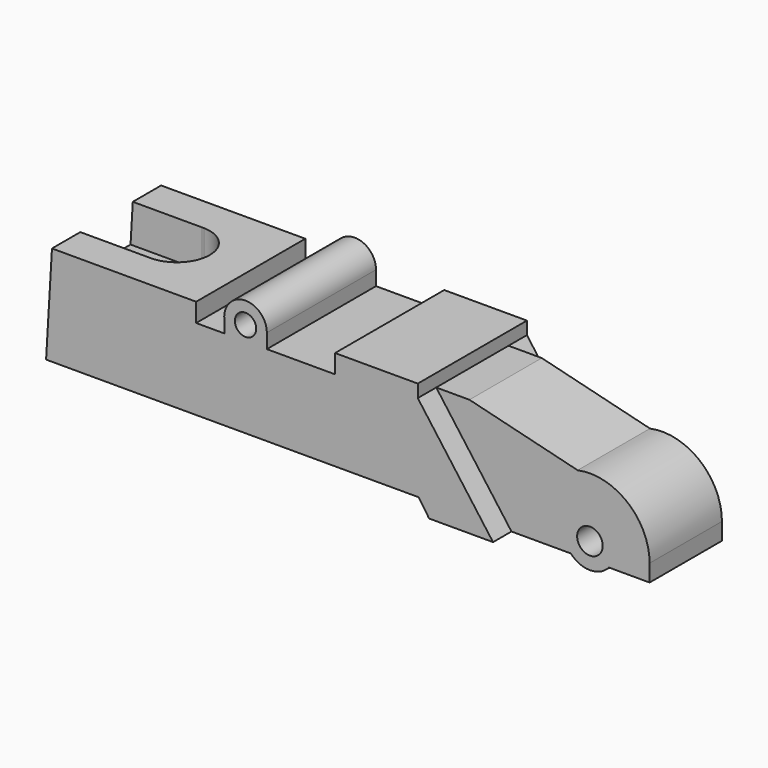
from build123d import *

# Parameters (mm, degrees)
F1_DEPTH  = 16
F2_R      = 1.5
F2_R_2    = 1.25
F3_DEPTH  = 16.001
F5_DEPTH  = 2.7
F8_DEPTH  = 14.501
F9_DEPTH  = 25
F11_DEPTH = 4.5


# Not quite as in the source:
# - a pattern or mirror of a feature is missing from the dataset's text; its kind, count and spacing are read off the source's solid


with BuildPart() as f1:
    # F0 (on Front) → F1 (new body)
    with BuildSketch(Plane.XZ):
        with BuildLine():
            Line((0.6909776407, 11.7), (0, 0))
            Line((0, 0), (43.7, 0))
            Line((43.7, 0), (44.92, -1.8))
            Line((44.92, -1.8), (59.3839320225, -1.8))
            ThreePointArc((59.3839320225, -1.8), (61.62, -2.8), (63.8560679775, -1.8))
            Line((63.8560679775, -1.8), (68.62, -1.8))
            Line((68.62, -1.8), (68.62, 0.2))
            ThreePointArc((68.62, 0.2), (66.0308120163, 5.6355070929), (60.1786464695, 7.05))
            Line((60.1786464695, 7.05), (47.4909776407, 10.2))
            Line((47.4909776407, 10.2), (43.5909776407, 10.2))
            Line((43.5909776407, 10.2), (43.5909776407, 11.7))
            Line((43.5909776407, 11.7), (33.8909776407, 11.7))
            Line((33.8909776407, 11.7), (33.8909776407, 9.5))
            Line((33.8909776407, 9.5), (25.8909776407, 9.5))
            Line((25.8909776407, 9.5), (25.8909776407, 11.2))
            ThreePointArc((25.8909776407, 11.2), (23.2847799515, 13.6977433917), (20.9, 10.9877963389))
            Line((20.9, 10.9877963389), (20.9, 9.5))
            Line((20.9, 9.5), (17.6, 9.5))
            Line((17.6, 9.5), (17.6, 11.7))
            Line((17.6, 11.7), (0.6909776407, 11.7))
        make_face()
    extrude(amount=F1_DEPTH)

    # F2 (on face) → F3 (cut, through all)
    with BuildSketch(Plane.XZ.offset(16)):
        with Locations((61.62, 0.2)):
            Circle(F2_R)
        with Locations((23.3909776407, 11.2)):
            Circle(F2_R_2)
    extrude(amount=-F3_DEPTH, mode=Mode.SUBTRACT)

    # F4 (on face) → F5 (cut)
    with BuildSketch(Plane.XZ.offset(16)):
        Polygon((69.0573006868, 10.2), (43.5909776407, 10.2), (52.42, -1.8), (58.7147176266, -4.3849991634), (70.332378149, -4.3849991634), align=None)
    f5 = extrude(amount=-F5_DEPTH, mode=Mode.SUBTRACT)

    # F5_copies: F5 across plane
    add(f5.mirror(Plane.ZX.offset(-8)), mode=Mode.SUBTRACT)

    # F7 (on face) → F8 (cut, through all)
    with BuildSketch(Plane.XY.offset(11.7)):
        with BuildLine():
            Line((8.9409776407, -5.75), (0.6909776407, -5.75))
            Line((0.6909776407, -5.75), (0.6909776407, -10.25))
            Line((0.6909776407, -10.25), (8.9409776407, -10.25))
            ThreePointArc((8.9409776407, -10.25), (11.1909776407, -8), (8.9409776407, -5.75))
        make_face()
    extrude(amount=-F8_DEPTH, mode=Mode.SUBTRACT)

    # F7 (on face) → F9 (cut)
    with BuildSketch(Plane.XY.offset(11.7)):
        with BuildLine():
            Line((8.9409776407, -5.75), (0.6909776407, -5.75))
            Line((0.6909776407, -5.75), (-0.8989692941, -5.75))
            Line((-0.8989692941, -5.75), (-0.8989692941, -10.25))
            Line((-0.8989692941, -10.25), (0.6909776407, -10.25))
            Line((0.6909776407, -10.25), (8.9409776407, -10.25))
            ThreePointArc((8.9409776407, -10.25), (11.1909776407, -8), (8.9409776407, -5.75))
        make_face()
    extrude(amount=-F9_DEPTH, mode=Mode.SUBTRACT)

    # F10 (on face) → F11 (cut)
    with BuildSketch(Plane.XY.offset(11.7)):
        with BuildLine():
            ThreePointArc((9.0590238842, -11.8481898452), (11.7047592925, -10.6803005393), (12.7909776407, -8))
            ThreePointArc((12.7909776407, -8), (11.7048621847, -5.3198055617), (9.0593193409, -4.1518192296))
            Line((9.0593193409, -4.1518192296), (8.8226359404, -4.1518192296))
            ThreePointArc((8.8226359404, -4.1518192296), (5.0909776435, -8.000147798), (8.8229313971, -11.8481898452))
            Line((8.8229313971, -11.8481898452), (9.0590238842, -11.8481898452))
        make_face()
        with BuildLine():
            Line((8.8226359404, -4.1518192296), (9.0593193409, -4.1518192296))
            ThreePointArc((9.0593193409, -4.1518192296), (8.9409776407, -4.15), (8.8226359404, -4.1518192296))
        make_face()
        with BuildLine():
            ThreePointArc((8.8229313971, -11.8481898452), (8.9409776407, -11.85), (9.0590238842, -11.8481898452))
            Line((9.0590238842, -11.8481898452), (8.8229313971, -11.8481898452))
        make_face()
        with BuildLine():
            ThreePointArc((8.8229313971, -11.8481898452), (5.0909776435, -8.000147798), (8.8226359404, -4.1518192296))
            Line((8.8226359404, -4.1518192296), (-1.5180813544, -4.1518192296))
            Line((-1.5180813544, -4.1518192296), (-2.6164921116, -11.8481898452))
            Line((-2.6164921116, -11.8481898452), (8.8229313971, -11.8481898452))
        make_face()
    extrude(amount=-F11_DEPTH, mode=Mode.SUBTRACT)


solid = f1.part
